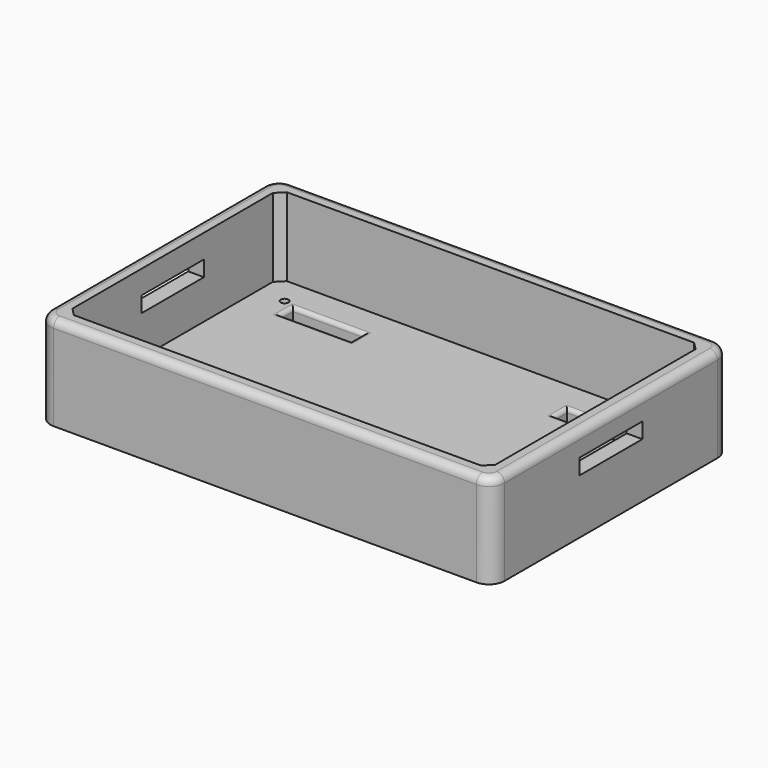
from build123d import *

# Parameters (mm, degrees)
F0_W      = 58
F0_H      = 38
F1_DEPTH  = 2
F2_W      = 58
F2_H      = 38
F2_W_2    = 54
F2_H_2    = 34
F3_DEPTH  = 10
F5_W      = 9
F5_H      = 2
F6_DEPTH  = 12.5
F7_R      = 2
F8_R      = 0.5
F9_R      = 1
F10_W     = 10
F10_H     = 2
F11_DEPTH = 58.0010001
F12_SIZE  = 1
F14_R     = 0.5
F15_DEPTH = 25


with BuildPart() as f1:
    # F0 (on Top) → F1 (new body)
    with BuildSketch(Plane.XY):
        with Locations((-18.2900002897, -8.8110647003)):
            Rectangle(F0_W, F0_H)
    extrude(amount=F1_DEPTH)

    # F2 (on face) → F3 (join)
    with BuildSketch(Plane.XY.offset(2)):
        with Locations((-18.2900002897, -8.8110647003)):
            Rectangle(F2_W, F2_H)
        with Locations((-18.2900002897, -8.8110647003)):
            Rectangle(F2_W_2, F2_H_2, mode=Mode.SUBTRACT)
    extrude(amount=F3_DEPTH)

    # F5 (on Top) → F6 (cut, symmetric)
    with BuildSketch(Plane.XY):
        with Locations((-35.7900002897, -20.8110647003)):
            Rectangle(F5_W, F5_H)
        with Locations((-35.7900002897, 3.1889352997)):
            Rectangle(F5_W, F5_H)
        with Locations((-0.7900002897, 3.1889352997)):
            Rectangle(F5_W, F5_H)
        with Locations((-0.7900002897, -20.8110647003)):
            Rectangle(F5_W, F5_H)
    extrude(amount=F6_DEPTH, both=True, mode=Mode.SUBTRACT)

    # F7
    f7_edges = [f1.edges().sort_by_distance(p)[0] for p in [
        (-47.29, -27.811065, 6),
        (10.71, -27.811065, 6),
        (10.71, 10.188935, 6),
        (-47.29, 10.188935, 6),
    ]]
    fillet(f7_edges, radius=F7_R)

    # F8
    f8_edges = [f1.edges().sort_by_distance(p)[0] for p in [
        (-0.79, 2.188935, 2),
        (-0.79, 4.188935, 2),
        (3.71, 3.188935, 2),
        (-5.29, 3.188935, 2),
        (-35.79, 2.188935, 2),
        (-35.79, 4.188935, 2),
        (-31.29, 3.188935, 2),
        (-40.29, 3.188935, 2),
        (-35.79, -19.811065, 2),
        (-35.79, -21.811065, 2),
        (-40.29, -20.811065, 0),
        (-31.29, -20.811065, 2),
        (-40.29, -20.811065, 2),
        (-0.79, -21.811065, 2),
        (-0.79, -19.811065, 2),
        (-5.29, -20.811065, 2),
        (3.71, -20.811065, 2),
    ]]
    fillet(f8_edges, radius=F8_R)

    # F9
    f9_edges = [f1.edges().sort_by_distance(p)[0] for p in [
        (-47.29, -8.811065, 12),
        (-18.29, -27.811065, 12),
        (10.71, -8.811065, 12),
        (-18.29, 10.188935, 12),
        (10.124213, 9.603149, 12),
        (-46.704214, 9.603149, 12),
        (10.124213, -27.225278, 12),
        (-46.704214, -27.225278, 12),
    ]]
    fillet(f9_edges, radius=F9_R)

    # F10 (on face) → F11 (cut, through all)
    with BuildSketch(Plane.YZ.offset(10.7099997103)):
        with Locations((-8.8110647003, 8)):
            Rectangle(F10_W, F10_H)
    extrude(amount=-F11_DEPTH, mode=Mode.SUBTRACT)

    # F12
    f12_edges = [f1.edges().sort_by_distance(p)[0] for p in [
        (-45.29, 8.188935, 7),
        (8.71, 8.188935, 7),
        (-45.29, -25.811065, 7),
        (8.71, -25.811065, 7),
    ]]
    chamfer(f12_edges, length=F12_SIZE)

    # F14 (on face) → F15 (cut)
    with BuildSketch(Plane.XY.offset(2)):
        with Locations((-41.7900002897, 4.6889352997)):
            Circle(F14_R)
        with Locations((5.2099997103, 3.1889352997)):
            Circle(F14_R)
        with Locations((5.2099997103, -17.8110647003)):
            Circle(F14_R)
    extrude(amount=-F15_DEPTH, mode=Mode.SUBTRACT)


solid = f1.part
